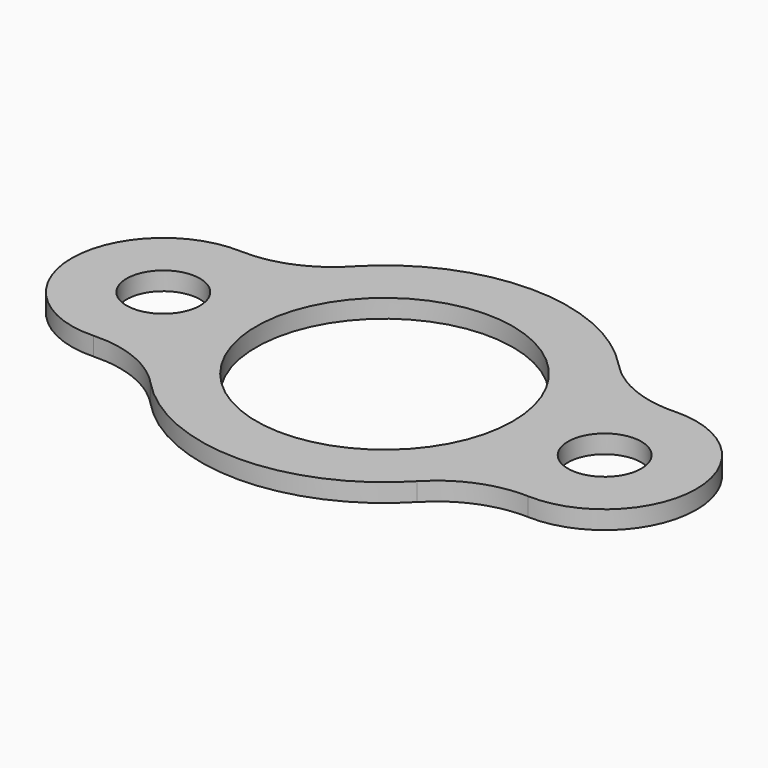
from build123d import *

# Parameters (mm, degrees)
F0_R     = 12.7
F0_R_2   = 44.45
F1_DEPTH = 6.35
F2_R     = 38.1


with BuildPart() as f1:
    # F0 (on Top) → F1 (new body)
    with BuildSketch(Plane.XY):
        with BuildLine():
            ThreePointArc((-58.0380028326, -25.7650970735), (-63.5, 0), (-58.0380028326, 25.7650970735))
            ThreePointArc((-58.0380028326, 25.7650970735), (-108.3412309289, 0), (-58.0380028326, -25.7650970735))
        make_face()
        with Locations((-76.5912309289, 0)):
            Circle(F0_R, mode=Mode.SUBTRACT)
        with BuildLine():
            ThreePointArc((57.94375, -25.976370723), (62.0954029096, -13.2819779212), (63.5, 0))
            ThreePointArc((63.5, 0), (62.0954029096, 13.2819779212), (57.94375, 25.976370723))
            ThreePointArc((57.94375, 25.976370723), (-0.1156721136, 63.4998946453), (-58.0380028326, 25.7650970735))
            ThreePointArc((-58.0380028326, 25.7650970735), (-63.5, 0), (-58.0380028326, -25.7650970735))
            ThreePointArc((-58.0380028326, -25.7650970735), (-0.1156721136, -63.4998946453), (57.94375, -25.976370723))
        make_face()
        Circle(F0_R_2, mode=Mode.SUBTRACT)
        with BuildLine():
            ThreePointArc((57.94375, 25.976370723), (62.0954029096, 13.2819779212), (63.5, 0))
            ThreePointArc((63.5, 0), (62.0954029096, -13.2819779212), (57.94375, -25.976370723))
            ThreePointArc((57.94375, -25.976370723), (107.95, 0), (57.94375, 25.976370723))
        make_face()
        with BuildLine():
            ThreePointArc((63.5, 0), (76.2, 12.7), (88.9, 0))
            ThreePointArc((88.9, 0), (76.2, -12.7), (63.5, 0))
        make_face(mode=Mode.SUBTRACT)
    extrude(amount=F1_DEPTH)

    # F2
    f2_edges = [f1.edges().sort_by_distance(p)[0] for p in [
        (-58.038003, 25.765097, 3.175),
        (57.94375, -25.976371, 3.175),
        (-58.038003, -25.765097, 3.175),
        (57.94375, 25.976371, 3.175),
    ]]
    fillet(f2_edges, radius=F2_R)


solid = f1.part
